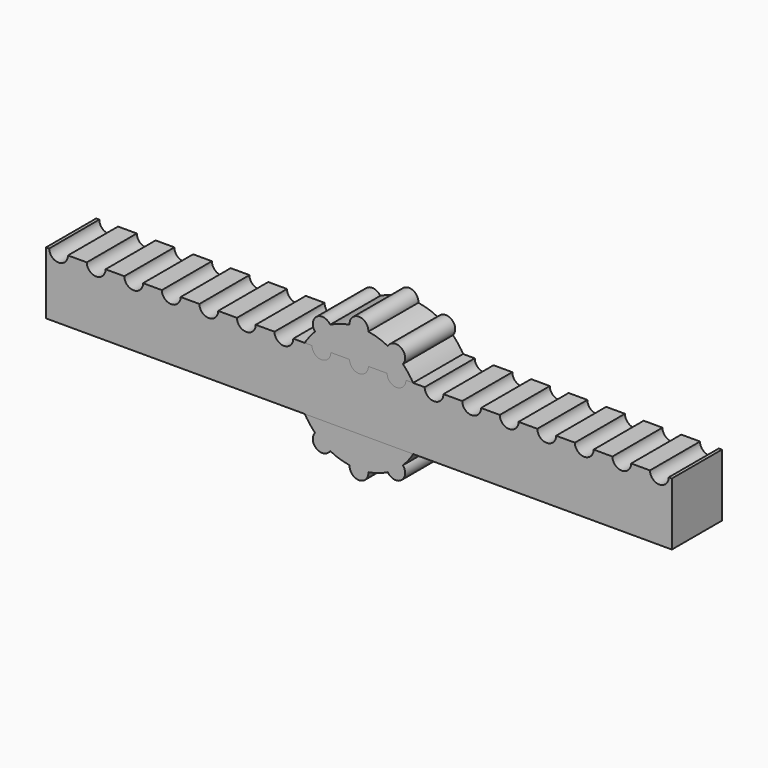
from build123d import *

# Parameters (mm, degrees)
F0_R     = 5
F2_DEPTH = 5
F1_R     = 0.75
F3_DEPTH = 5
F4_W     = 50
F4_H     = 5
F5_DEPTH = 5
F6_R     = 0.75
F7_DEPTH = 5


with BuildPart() as f2:
    # F0 (on Front) → F2 (new body)
    with BuildSketch(Plane.XZ):
        Circle(F0_R)
    extrude(amount=F2_DEPTH)

    # F1 (on Front) → F3 (join)
    with BuildSketch(Plane.XZ):
        with Locations((0, 5)):
            Circle(F1_R)
        with Locations((-2.9389262615, 4.0450849719)):
            Circle(F1_R)
        with Locations((-4.7552825815, 1.5450849719)):
            Circle(F1_R)
        with Locations((-4.7552825815, -1.5450849719)):
            Circle(F1_R)
        with Locations((-2.9389262615, -4.0450849719)):
            Circle(F1_R)
        with Locations((0, -5)):
            Circle(F1_R)
        with Locations((2.9389262615, -4.0450849719)):
            Circle(F1_R)
        with Locations((4.7552825815, -1.5450849719)):
            Circle(F1_R)
        with Locations((4.7552825815, 1.5450849719)):
            Circle(F1_R)
        with Locations((2.9389262615, 4.0450849719)):
            Circle(F1_R)
    extrude(amount=F3_DEPTH)


with BuildPart() as f5:
    # F4 (on Front) → F5 (new body)
    with BuildSketch(Plane.XZ):
        Rectangle(F4_W, F4_H)
    extrude(amount=F5_DEPTH)

    # F6 (on Front) → F7 (cut)
    with BuildSketch(Plane.XZ):
        with Locations((-24, 2.5)):
            Circle(F6_R)
        with Locations((-21, 2.5)):
            Circle(F6_R)
        with Locations((-18, 2.5)):
            Circle(F6_R)
        with Locations((-15, 2.5)):
            Circle(F6_R)
        with Locations((-12, 2.5)):
            Circle(F6_R)
        with Locations((-9, 2.5)):
            Circle(F6_R)
        with Locations((-6, 2.5)):
            Circle(F6_R)
        with Locations((-3, 2.5)):
            Circle(F6_R)
        with Locations((0, 2.5)):
            Circle(F6_R)
        with Locations((3, 2.5)):
            Circle(F6_R)
        with Locations((6, 2.5)):
            Circle(F6_R)
        with Locations((9, 2.5)):
            Circle(F6_R)
        with Locations((12, 2.5)):
            Circle(F6_R)
        with Locations((15, 2.5)):
            Circle(F6_R)
        with Locations((18, 2.5)):
            Circle(F6_R)
        with Locations((21, 2.5)):
            Circle(F6_R)
        with Locations((24, 2.5)):
            Circle(F6_R)
    extrude(amount=F7_DEPTH, mode=Mode.SUBTRACT)


solid = Compound([f2.part, f5.part])
